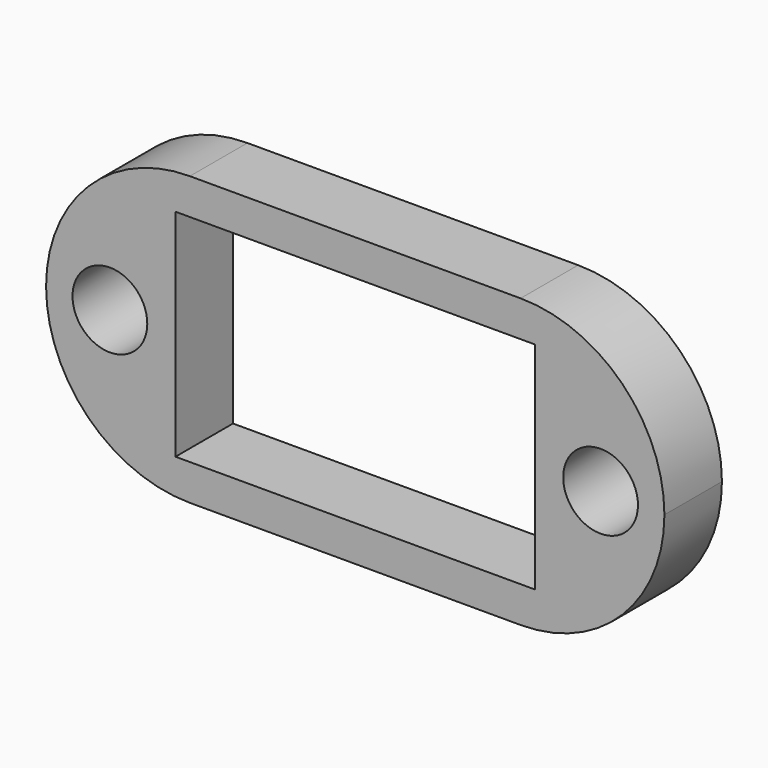
from build123d import *

# Parameters (mm, degrees)
F0_W     = 86
F0_H     = 40
F1_DEPTH = 10
F2_R     = 5.2
F3_DEPTH = 25
F4_W     = 50
F4_H     = 30
F5_DEPTH = 25
F6_R     = 19.99999


# Not quite as in the source:
# - a fillet or chamfer is up to 0.001 mm smaller than in the source, because OpenCascade refuses the exact size


with BuildPart() as f1:
    # F0 (on Front) → F1 (new body)
    with BuildSketch(Plane.XZ):
        Rectangle(F0_W, F0_H)
    extrude(amount=-F1_DEPTH)

    # F2 (on face) → F3 (cut)
    with BuildSketch(Plane.XZ):
        with Locations((-34.125, 0)):
            Circle(F2_R)
        with Locations((34.125, 0)):
            Circle(F2_R)
    extrude(amount=-F3_DEPTH, mode=Mode.SUBTRACT)

    # F4 (on face) → F5 (cut)
    with BuildSketch(Plane.XZ):
        Rectangle(F4_W, F4_H)
    extrude(amount=-F5_DEPTH, mode=Mode.SUBTRACT)

    # F6 (radius 20 in the source; OpenCascade refuses exactly that, so slightly less here)
    f6_edges = [f1.edges().sort_by_distance(p)[0] for p in [
        (-43, 5, 20),
        (43, 5, 20),
        (43, 5, -20),
        (-43, 5, -20),
    ]]
    fillet(f6_edges, radius=F6_R)


solid = f1.part
